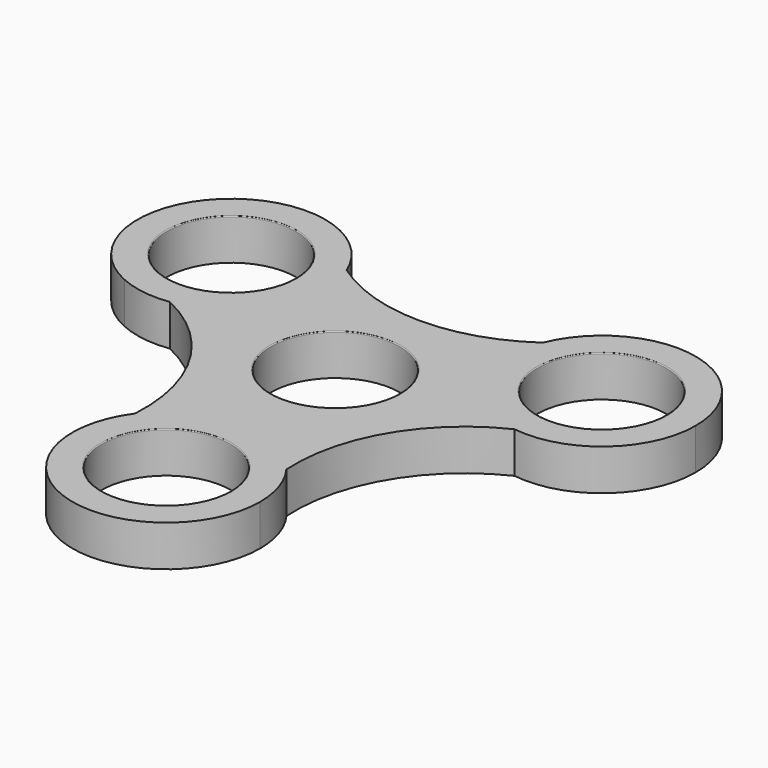
from build123d import *

# Parameters (mm, degrees)
F0_R     = 11
F1_DEPTH = 7
F2_DEPTH = 7
F3_R     = 0.15
F4_R     = 0.15
F5_R     = 0.15


# Not quite as in the source:
# - a feature names something its author has since deleted; it is built from what else it names


with BuildPart() as f1:
    # F0 (on Top) → F1 (new body)
    with BuildSketch(Plane.XY):
        with BuildLine():
            ThreePointArc((29.3501442774, 1.4728811124), (17.7035935394, 9.3195381001), (16.7314646223, 23.3290753994))
            ThreePointArc((16.7314646223, 23.3290753994), (0, 18.0157402468), (-16.7314646223, 23.3290753994))
            ThreePointArc((-16.7314646223, 23.3290753994), (-15.8555966996, 20.3808641164), (-15.56, 17.3195381001))
            ThreePointArc((-15.56, 17.3195381001), (-19.4902507988, 6.8161503505), (-29.3501442774, 1.4728811124))
            ThreePointArc((-29.3501442774, 1.4728811124), (-16.8351135056, -10.0081099666), (-12.8952216464, -26.5282916699))
            ThreePointArc((-12.8952216464, -26.5282916699), (-0.0001071921, -20.0000000004), (12.8950947338, -26.5281188876))
            ThreePointArc((12.8950947338, -26.5281188876), (16.8350899961, -10.0080120701), (29.3501442774, 1.4728811124))
        make_face()
        Circle(F0_R, mode=Mode.SUBTRACT)
    extrude(amount=F1_DEPTH)

    # F0 (on Top) → F2 (join)
    with BuildSketch(Plane.XY):
        with BuildLine():
            ThreePointArc((29.3501442774, 1.4728811124), (42.0633877496, 5.2497888988), (47.56, 17.3195381001))
            ThreePointArc((47.56, 17.3195381001), (34.6213260163, 33.0239414005), (16.7314646223, 23.3290753994))
            ThreePointArc((16.7314646223, 23.3290753994), (17.7035935394, 9.3195381001), (29.3501442774, 1.4728811124))
        make_face()
        with Locations((31.56, 17.3195381001)):
            Circle(F0_R, mode=Mode.SUBTRACT)
        with BuildLine():
            ThreePointArc((-15.56, 17.3195381001), (-15.8555966996, 20.3808641164), (-16.7314646223, 23.3290753994))
            ThreePointArc((-16.7314646223, 23.3290753994), (-42.6554805123, 28.8473441446), (-38.1316823001, 2.7314267848))
            ThreePointArc((-38.1316823001, 2.7314267848), (-33.8298826127, 1.4813679746), (-29.3501442774, 1.4728811124))
            ThreePointArc((-29.3501442774, 1.4728811124), (-19.4902507988, 6.8161503505), (-15.56, 17.3195381001))
        make_face()
        with Locations((-31.56, 17.3195381001)):
            Circle(F0_R, mode=Mode.SUBTRACT)
        with BuildLine():
            ThreePointArc((16, -36), (15.2039717794, -31.0161017135), (12.8950947338, -26.5281188876))
            ThreePointArc((12.8950947338, -26.5281188876), (-0.0001071921, -20.0000000004), (-12.8952216464, -26.5282916699))
            ThreePointArc((-12.8952216464, -26.5282916699), (-4.9837964273, -51.2040051687), (16, -36))
        make_face()
        with Locations((0, -36)):
            Circle(F0_R, mode=Mode.SUBTRACT)
    extrude(amount=F2_DEPTH)

    # F3
    f3_edges = [f1.edges().sort_by_distance(p)[0] for p in [
        (-11, 0, 7),
    ]]
    fillet(f3_edges, radius=F3_R)

    # F4
    f4_edges = [f1.edges().sort_by_distance(p)[0] for p in [
        (-42.56, 17.319538, 7),
        (-11, -36, 7),
    ]]
    fillet(f4_edges, radius=F4_R)

    # F5
    f5_edges = [f1.edges().sort_by_distance(p)[0] for p in [
        (20.56, 17.319538, 7),
    ]]
    fillet(f5_edges, radius=F5_R)


solid = f1.part
